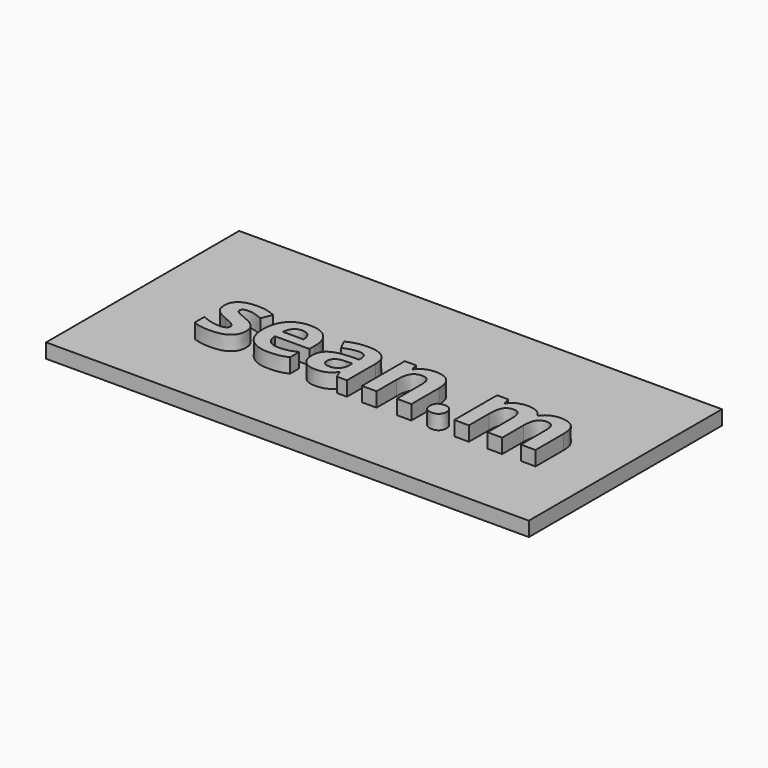
from build123d import *

# Parameters (mm, degrees)
F0_W         = 100
F0_H         = 50
F1_DEPTH     = 3
F2_TEXT_SIZE = 20.2963917723
F3_DEPTH     = 3


# Not quite as in the source:
# - Text() gives the source's letters only with a copy of the font that has no kerning and outlines rounded to 1/6400 em; it was checked with that copy


with BuildPart() as f1:
    # F0 (on Top) → F1 (new body)
    with BuildSketch(Plane.XY):
        with Locations((50, 25)):
            Rectangle(F0_W, F0_H)
    extrude(amount=F1_DEPTH)

    # F2 (on face) → F3 (join)
    with BuildSketch(Plane.XY.offset(3)):
        with Locations((17.1005148441, 15.515464358)):
            Text('sean.m', F2_TEXT_SIZE, font='Open Sans', font_style=FontStyle.BOLD, text_align=(TextAlign.LEFT, TextAlign.BOTTOM))
    extrude(amount=F3_DEPTH)


solid = f1.part
